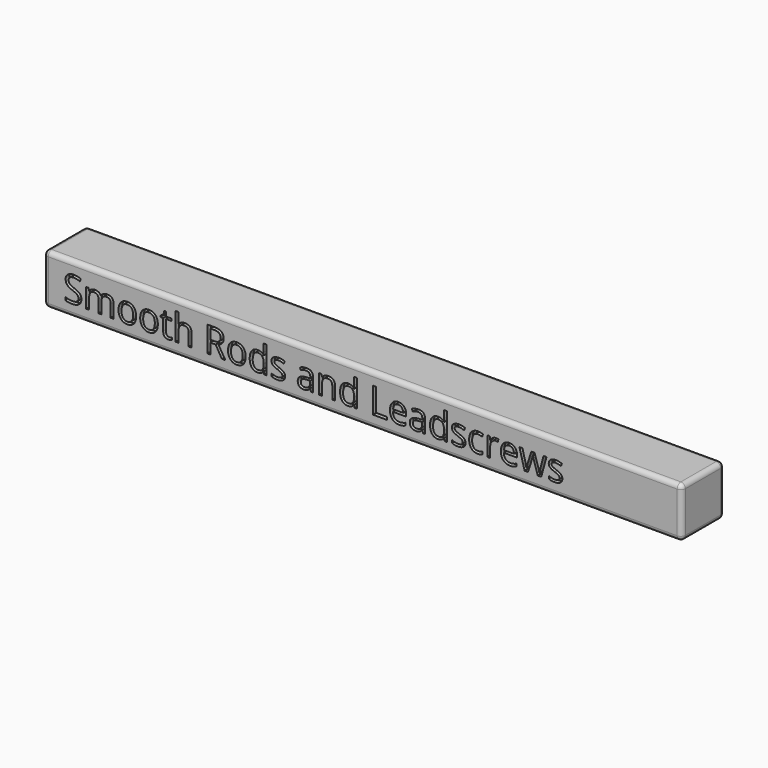
from build123d import *

# Parameters (mm, degrees)
F0_W         = 420
F0_H         = 35
F1_DEPTH     = 33
F2_R         = 3
F3_TEXT_SIZE = 23.6111111111
F4_DEPTH     = 3


# Not quite as in the source:
# - Text() gives the source's letters only with a copy of the font that has no kerning and outlines rounded to 1/6400 em; it was checked with that copy


with BuildPart() as f1:
    # F0 (on Top) → F1 (new body)
    with BuildSketch(Plane.XY):
        with Locations((-210, 17.5)):
            Rectangle(F0_W, F0_H)
    extrude(amount=F1_DEPTH)

    # F2
    f2_edges = [f1.edges().sort_by_distance(p)[0] for p in [
        (-420, 0, 16.5),
        (0, 0, 16.5),
        (-210, 0, 0),
        (-210, 0, 33),
        (0, 17.5, 33),
        (-210, 35, 33),
        (-420, 17.5, 33),
        (0, 35, 16.5),
        (0, 17.5, 0),
        (-420, 35, 16.5),
        (-210, 35, 0),
        (-420, 17.5, 0),
    ]]
    fillet(f2_edges, radius=F2_R)

    # F3 (on face) → F4 (cut)
    with BuildSketch(Plane.XZ):
        with Locations((-407, 8)):
            Text('Smooth Rods and Leadscrews', F3_TEXT_SIZE, font='Open Sans', text_align=(TextAlign.LEFT, TextAlign.BOTTOM))
    extrude(amount=-F4_DEPTH, mode=Mode.SUBTRACT)


solid = f1.part
